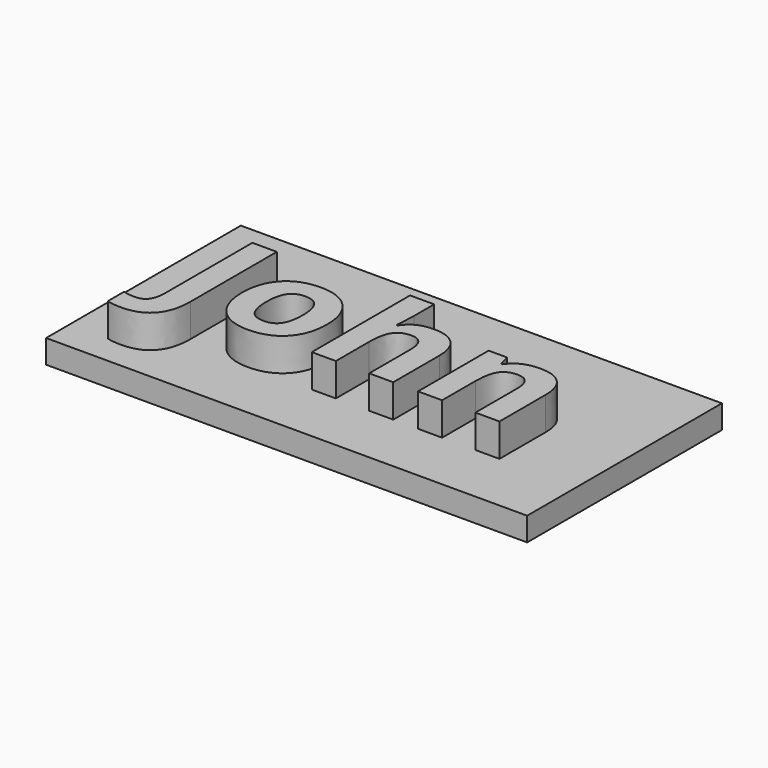
from build123d import *

# Parameters (mm, degrees)
F0_W         = 102.2350043058
F0_H         = 51.7398025841
F1_DEPTH     = 5
F2_TEXT_SIZE = 34.3554988928
F3_DEPTH     = 7


# Not quite as in the source:
# - Text() gives the source's letters only with a copy of the font that has no kerning and outlines rounded to 1/6400 em; it was checked with that copy


with BuildPart() as f1:
    # F0 (on Top) → F1 (new body)
    with BuildSketch(Plane.XY):
        with Locations((3.3782012761, 15.113000758)):
            Rectangle(F0_W, F0_H)
    extrude(amount=F1_DEPTH)

    # F2 (on face) → F3 (join)
    with BuildSketch(Plane.XY.offset(5)):
        with Locations((-37.0670903015, 2.3192008215)):
            Text('John', F2_TEXT_SIZE, font='Open Sans', font_style=FontStyle.BOLD, text_align=(TextAlign.LEFT, TextAlign.BOTTOM))
    extrude(amount=F3_DEPTH)


solid = f1.part
